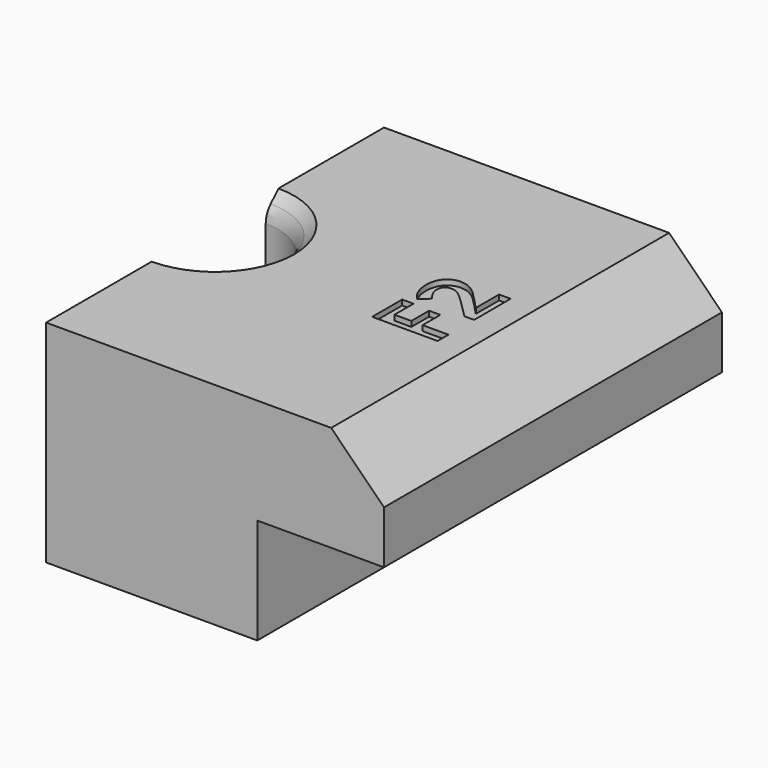
from build123d import *

# Parameters (mm, degrees)
F1_DEPTH     = 40
F2_R         = 1.65
F3_DEPTH     = 8
F6_T2_ANGLE  = 180
F6_T4_ANGLE  = 180
F7_R         = 2
F8_TEXT_SIZE = 8.6744375169
F9_DEPTH     = 0.5


# Not quite as in the source:
# - a fillet or chamfer that OpenCascade refuses, or shapes differently, is made with other operations: its cross-section is extruded or revolved along the edge and cut away or added
# - Text() gives the source's letters only with a copy of the font that has no kerning and outlines rounded to 1/6400 em; it was checked with that copy


with BuildPart() as f1:
    # F0 (on Front) → F1 (new body)
    with BuildSketch(Plane.XZ):
        Polygon((0, -10), (0, 0), (12, 0), (12, 5), (7, 10), (-20, 10), (-20, -10), align=None)
    extrude(amount=F1_DEPTH)

    # F2 (on face) → F3 (cut)
    with BuildSketch(Plane(origin=(0, 0, 0), x_dir=(1, 0, 0), z_dir=(0, 0, -1))):
        with Locations((5, 32.5)):
            Circle(F2_R)
        with Locations((5, 7.5)):
            Circle(F2_R)
    extrude(amount=-F3_DEPTH, mode=Mode.SUBTRACT)

    # F4 (on face) → F5 (revolve, cut)
    with BuildSketch(Plane(origin=(-20, 0, 0), x_dir=(0, -1, 0), z_dir=(-1, 0, 0))):
        Polygon((20, -10), (20, 10), (12.5, 10), (14, 8.5), (14, 0.5), (14.25, 0.5), (16.25, -1.5), (16.25, -2), (13.5, -2), (13.5, -10), align=None)
    revolve(axis=Axis((-20, -20, 0), (0, 0, -1)), mode=Mode.SUBTRACT)

    # F6: fillet of radius 0.5 on 2 edges, made by hand

    # F6_s1 → F6_t2 (revolve)
    with BuildSketch(Plane.YZ.offset(-20)):
        with BuildLine():
            ThreePointArc((-13.5, -2.5), (-13.6464466094, -2.1464466094), (-14, -2))
            Line((-14, -2), (-14, -1.99))
            Line((-14, -1.99), (-13.49, -1.99))
            Line((-13.49, -1.99), (-13.49, -2.5))
            Line((-13.49, -2.5), (-13.5, -2.5))
        make_face()
    revolve(axis=Axis((-20, -20, -2), (0, 0, -1)), revolution_arc=F6_T2_ANGLE)

    # F6_s3 → F6_t4 (revolve)
    with BuildSketch(Plane.YZ.offset(-20)):
        with BuildLine():
            ThreePointArc((-14, 0.9330127019), (-14.0669872981, 0.6830127019), (-14.25, 0.5))
            Line((-14.25, 0.5), (-14.245, 0.491339746))
            ThreePointArc((-14.245, 0.491339746), (-14.125, 0.49), (-14, 0.49))
            Line((-14, 0.49), (-13.99, 0.5))
            Line((-13.99, 0.5), (-13.99, 0.9330127019))
            Line((-13.99, 0.9330127019), (-14, 0.9330127019))
        make_face()
    revolve(axis=Axis((-20, -20, 0.5), (0, 0, -1)), revolution_arc=F6_T4_ANGLE)

    # F7
    f7_edges = [f1.edges().sort_by_distance(p)[0] for p in [
        (-14, -20, 8.5),
    ]]
    fillet(f7_edges, radius=F7_R)

    # F8 (on face) → F9 (cut)
    with BuildSketch(Plane.XY.offset(10)):
        with Locations(Location((4.4465429643, -25), (0, 0, 90))):
            Text('F2', F8_TEXT_SIZE, font='Open Sans', font_style=FontStyle.BOLD, text_align=(TextAlign.LEFT, TextAlign.BOTTOM))
    extrude(amount=-F9_DEPTH, mode=Mode.SUBTRACT)


solid = f1.part
